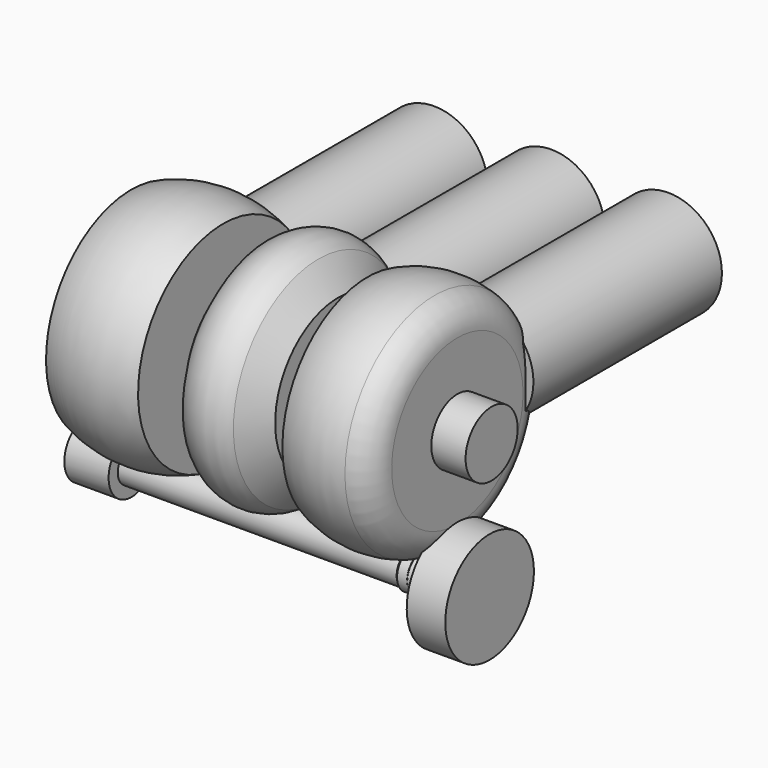
from build123d import *

# Parameters (mm, degrees)
F5_W      = 33
F5_H      = 22.8
F5_W_2    = 17.596
F5_W_3    = 20.673
F5_W_4    = 24
F4_R      = 37.5
F9_DEPTH  = 165
F12_DEPTH = 100
F13_W     = 196.8
F13_H     = 12
F15_SIZE  = 0.49999
F16_SIZE  = 1.49999


# Not quite as in the source:
# - a fillet or chamfer is up to 0.001 mm smaller than in the source, because OpenCascade refuses the exact size


with BuildPart() as f6:
    # F5 (on Top) → F6 (revolve)
    with BuildSketch(Plane.XY):
        with Locations((-48.725, 11.4)):
            Rectangle(F5_W, F5_H)
        with BuildLine():
            Line((-32.225, 22.8), (-32.225, 0))
            Line((-32.225, 0), (32.232, 0))
            Line((32.232, 0), (32.232, 22.8))
            Line((32.232, 22.8), (32.232, 74.5))
            ThreePointArc((32.232, 74.5), (0.0035, 81), (-32.225, 74.5))
            Line((-32.225, 74.5), (-32.225, 22.8))
        make_face()
        with Locations((41.03, 11.4)):
            Rectangle(F5_W_2, F5_H)
        with BuildLine():
            Line((49.828, 22.8), (49.828, 0))
            Line((49.828, 0), (112.63, 0))
            Line((112.63, 0), (112.63, 22.8))
            Line((112.63, 22.8), (112.63, 55))
            Line((112.63, 55), (98.9759530049, 74.5))
            ThreePointArc((98.9759530049, 74.5), (81.229, 81), (63.4820469951, 74.5))
            Line((63.4820469951, 74.5), (49.828, 55))
            Line((49.828, 55), (49.828, 22.8))
        make_face()
        with Locations((122.9665, 11.4)):
            Rectangle(F5_W_3, F5_H)
        with BuildLine():
            Line((133.303, 22.8), (133.303, 0))
            Line((133.303, 0), (196.225, 0))
            Line((196.225, 0), (196.225, 22.8))
            Line((196.225, 22.8), (196.225, 57.5))
            ThreePointArc((196.225, 57.5), (191.7945491151, 70.6775352134), (180.303, 78.5018964191))
            ThreePointArc((180.303, 78.5018964191), (156.4405623285, 80.7575727631), (133.303, 74.5))
            Line((133.303, 74.5), (133.303, 22.8))
        make_face()
        with Locations((208.225, 11.4)):
            Rectangle(F5_W_4, F5_H)
    revolve(axis=Axis((36.7081814394, 0, 0), (1, 0, 0)))

    # F4 (on offset) → F9 (join)
    with BuildSketch(Plane.XZ.offset(-60)):
        with Locations((164, 7.5)):
            Circle(F4_R)
        with Locations((82, 7.5)):
            Circle(F4_R)
        with Locations((0, 7.5)):
            Circle(F4_R)
    extrude(amount=-F9_DEPTH)

    # F11 (on Front) → F12 (cut, symmetric)
    with BuildSketch(Plane.XZ):
        Polygon((-15.372583002, -80), (-38, -57.372583002), (-38, -80), align=None)
    extrude(amount=F12_DEPTH, both=True, mode=Mode.SUBTRACT)

    # F13 (on offset) → F14 (revolve)
    with BuildSketch(Plane.XY.offset(-95)):
        Polygon((191.8, 14), (191.8, 0), (218.8, 0), (218.8, 38.8), (191.8, 38.8), align=None)
        Polygon((172.3, 13.5), (172.3, 0), (191.8, 0), (191.8, 14), (172.3, 14), align=None)
        Polygon((164.8, 12), (164.8, 0), (172.3, 0), (172.3, 13.5), (164.8, 13.5), align=None)
        with Locations((66.4, 6)):
            Rectangle(F13_W, F13_H)
        Polygon((-63, 20), (-63, 0), (-32, 0), (-32, 12), (-32, 20), align=None)
    revolve(axis=Axis((109.8132303458, 0, -95), (1, 0, 0)))

    # F15 (size 0.5 in the source; OpenCascade refuses exactly that, so slightly less here)
    f15_edges = [f6.edges().sort_by_distance(p)[0] for p in [
        (172.3, -13.5, -95),
    ]]
    chamfer(f15_edges, length=F15_SIZE)

    # F16 (size 1.5 in the source; OpenCascade refuses exactly that, so slightly less here)
    f16_edges = [f6.edges().sort_by_distance(p)[0] for p in [
        (164.8, -12, -95),
    ]]
    chamfer(f16_edges, length=F16_SIZE)


solid = f6.part
